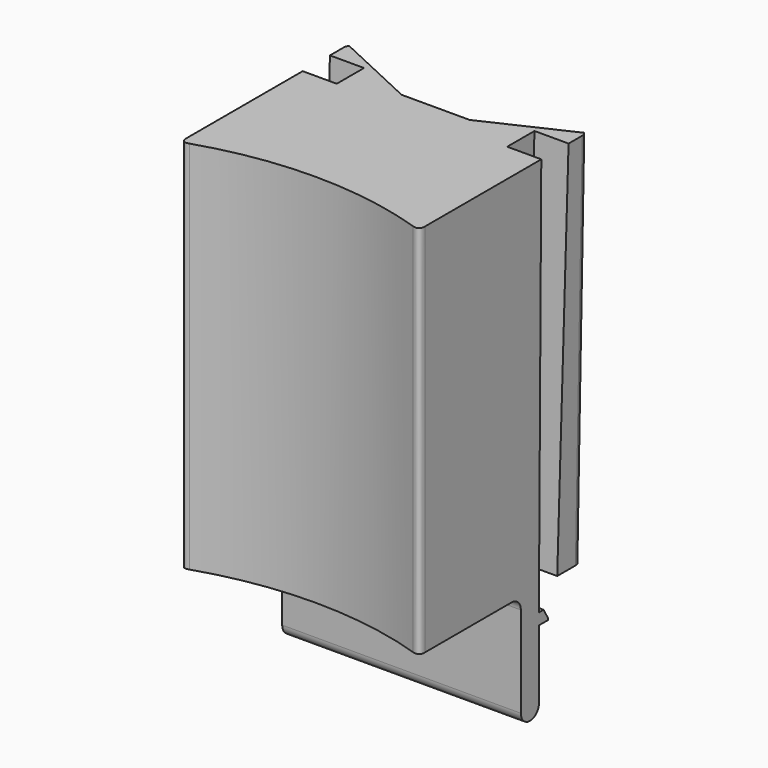
from build123d import *

# Parameters (mm, degrees)
F1_DEPTH    = 33
F3_DEPTH    = 21.001
F4_DEPTH    = 3
F6_T1_DEPTH = 35.508521627
F6_T3_DEPTH = 36.4826554363
F7_W        = 21
F7_H        = 2
F8_DEPTH    = 10
F9_W        = 21
F9_H        = 1
F10_DEPTH   = 1
F11_SIZE2   = 0.8660254038
F11_SIZE    = 0.5
F12_R       = 0.99999


# Not quite as in the source:
# - a fillet or chamfer that OpenCascade refuses, or shapes differently, is made with other operations: its cross-section is extruded or revolved along the edge and cut away or added
# - a fillet or chamfer is up to 0.001 mm smaller than in the source, because OpenCascade refuses the exact size
# - a pattern or mirror of a feature is missing from the dataset's text; its kind, count and spacing are read off the source's solid


with BuildPart() as f1:
    # F0 (on Top) → F1 (new body)
    with BuildSketch(Plane.XY):
        Polygon((-33.9465141296, 18.5), (-33.9465141296, 15), (-26.4407399079, 15), align=None)
        Polygon((-20.4522883514, 15), (-12.9465141296, 15), (-12.9465141296, 18.5), align=None)
        with BuildLine():
            Line((-33.9465141296, 15), (-33.9465141296, 0))
            ThreePointArc((-33.9465141296, 0), (-23.4465141296, 1.783504535), (-12.9465141296, 0))
            Line((-12.9465141296, 0), (-12.9465141296, 15))
            Line((-12.9465141296, 15), (-20.4522883514, 15))
            Line((-20.4522883514, 15), (-26.4407399079, 15))
            Line((-26.4407399079, 15), (-33.9465141296, 15))
        make_face()
    extrude(amount=F1_DEPTH)

    # F2 (on face) → F3 (cut, through all)
    with BuildSketch(Plane.YZ.offset(-12.9465141296)):
        Polygon((18.5, 0), (18.5, 33), (17.75, 0), align=None)
    extrude(amount=-F3_DEPTH, mode=Mode.SUBTRACT)

    # F2 (on face) → F4 (cut)
    with BuildSketch(Plane.YZ.offset(-12.9465141296)):
        Polygon((15.25, 0), (16.5, 33), (13.5, 33), (13.25, 0), align=None)
    f4 = extrude(amount=-F4_DEPTH, mode=Mode.SUBTRACT)

    # F4_copies: F4 across plane
    add(f4.mirror(Plane(origin=(-23.446514, 0, 0), x_dir=(0, 0, -1), z_dir=(-1, 0, 0))), mode=Mode.SUBTRACT)

    # F6: fillet of radius 0.5 on 4 edges, made by hand

    # F6_s2 → F6_t1 (cut)
    with BuildSketch(Plane(origin=(0, 0.7875654118, 34.6528781205), x_dir=(1, 0, 0), z_dir=(0, -0.0227214054, -0.9997418355))):
        with BuildLine():
            add(Edge.make_bspline(
                [(-13.4465141296, -17.7454175809), (-12.9465141296, -17.7454175809), (-12.9465141296, -17.2454175809)],
                knots=[0, 0, 0, 1, 1, 1], degree=2, weights=[1, 1, 1]))
            Line((-12.9465141296, -17.2454175809), (-12.9465141296, -17.7454175809))
            Line((-12.9465141296, -17.7454175809), (-13.4465141296, -17.7454175809))
        make_face()
        with BuildLine():
            add(Edge.make_bspline(
                [(-33.9465141296, -17.2454175809), (-33.9465141296, -17.7454175809), (-33.4465141296, -17.7454175809)],
                knots=[0, 0, 0, 1, 1, 1], degree=2, weights=[1, 1, 1]))
            Line((-33.4465141296, -17.7454175809), (-33.9465141296, -17.7454175809))
            Line((-33.9465141296, -17.7454175809), (-33.9465141296, -17.2454175809))
        make_face()
    extrude(amount=F6_T1_DEPTH, mode=Mode.SUBTRACT)

    # F6_s4 → F6_t3 (cut)
    with BuildSketch(Plane.XY.offset(-1.7413277182)):
        with BuildLine():
            add(Edge.make_bspline(
                [(-33.291715368, 0.2210972397), (-33.9465141296, 0.0078982049), (-33.9465141296, 0.6965310873)],
                knots=[0, 0, 0, 1, 1, 1], degree=2, weights=[1, 1, 1]))
            Line((-33.9465141296, 0.6965310873), (-33.9465141296, 0))
            ThreePointArc((-33.9465141296, 0), (-33.6197154132, 0.1123275396), (-33.291715368, 0.2210972397))
        make_face()
        with BuildLine():
            add(Edge.make_bspline(
                [(-12.9465141296, 0.6965310873), (-12.9465141296, 0.0078982049), (-13.6013128912, 0.2210972397)],
                knots=[0, 0, 0, 1, 1, 1], degree=2, weights=[1, 1, 1]))
            ThreePointArc((-13.6013128912, 0.2210972397), (-13.2733128461, 0.1123275396), (-12.9465141296, 0))
            Line((-12.9465141296, 0), (-12.9465141296, 0.6965310873))
        make_face()
    extrude(amount=F6_T3_DEPTH, mode=Mode.SUBTRACT)

    # F7 (on face) → F8 (join)
    with BuildSketch(Plane(origin=(0, 0, 0), x_dir=(1, 0, 0), z_dir=(0, 0, -1))):
        with Locations((-23.4465141296, -12.25)):
            Rectangle(F7_W, F7_H)
    extrude(amount=F8_DEPTH)

    # F9 (on face) → F10 (join)
    with BuildSketch(Plane(origin=(0, 13.25, 0), x_dir=(-1, 0, 0), z_dir=(0, 1, 0))):
        with Locations((23.4465141296, -2.5)):
            Rectangle(F9_W, F9_H)
    extrude(amount=F10_DEPTH)

    # F11
    f11_edges = [f1.edges().sort_by_distance(p)[0] for p in [
        (-23.446514, 14.25, -2),
    ]]
    f11_side = f1.faces().sort_by_distance((-23.446514, 13.75, -2))[0]
    chamfer(f11_edges, length=F11_SIZE, length2=F11_SIZE2, reference=f11_side)

    # F12 (radius 1 in the source; OpenCascade refuses exactly that, so slightly less here)
    f12_edges = [f1.edges().sort_by_distance(p)[0] for p in [
        (-23.446514, 11.25, 0),
        (-23.446514, 13.25, -10),
        (-23.446514, 11.25, -10),
    ]]
    fillet(f12_edges, radius=F12_R)


solid = f1.part
